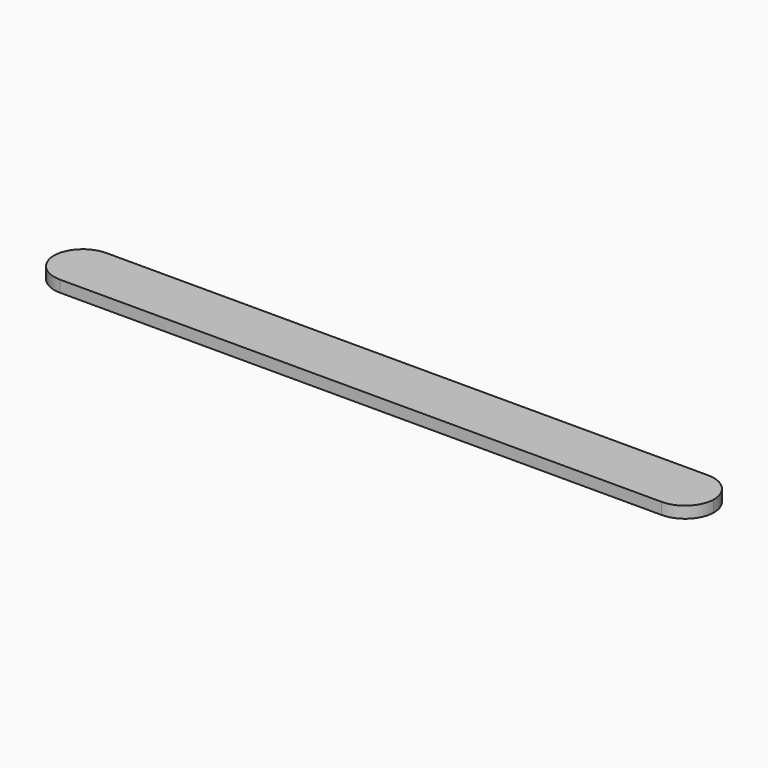
from build123d import *

# Parameters (mm, degrees)
F0_W        = 114.3
F0_H        = 10
F1_DEPTH    = 2
F2_R        = 5.08
F3_R        = 5.08
F4_T1_DEPTH = 27.3873984488
F5_T1_DEPTH = 27.3873984488


# Not quite as in the source:
# - a fillet or chamfer that OpenCascade refuses, or shapes differently, is made with other operations: its cross-section is extruded or revolved along the edge and cut away or added


with BuildPart() as f1:
    # F0 (on Top) → F1 (new body)
    with BuildSketch(Plane.XY):
        with Locations((-2.3567027405, -37.438484022)):
            Rectangle(F0_W, F0_H)
    extrude(amount=F1_DEPTH)

    # F2
    f2_edges = [f1.edges().sort_by_distance(p)[0] for p in [
        (-59.506703, -32.438484, 1),
    ]]
    fillet(f2_edges, radius=F2_R)

    # F3
    f3_edges = [f1.edges().sort_by_distance(p)[0] for p in [
        (54.793297, -32.438484, 1),
    ]]
    fillet(f3_edges, radius=F3_R)

    # F4: fillet of radius 5.08 on 1 edges, made by hand

    # F4_s2 → F4_t1 (cut)
    with BuildSketch(Plane.XY.offset(-12.6936992244)):
        with BuildLine():
            ThreePointArc((-59.5067027405, -37.518484022), (-57.9643043793, -41.0067164708), (-54.4292230507, -42.438484022))
            Line((-54.4292230507, -42.438484022), (-59.5067027405, -42.438484022))
            Line((-59.5067027405, -42.438484022), (-59.5067027405, -37.518484022))
        make_face()
    extrude(amount=F4_T1_DEPTH, mode=Mode.SUBTRACT)

    # F5: fillet of radius 5.08 on 1 edges, made by hand

    # F5_s2 → F5_t1 (cut)
    with BuildSketch(Plane.XY.offset(-12.6936992244)):
        with BuildLine():
            ThreePointArc((54.7932972595, -37.518484022), (53.2508988984, -41.0067164708), (49.7158175697, -42.438484022))
            Line((49.7158175697, -42.438484022), (54.7932972595, -42.438484022))
            Line((54.7932972595, -42.438484022), (54.7932972595, -37.518484022))
        make_face()
    extrude(amount=F5_T1_DEPTH, mode=Mode.SUBTRACT)


solid = f1.part
